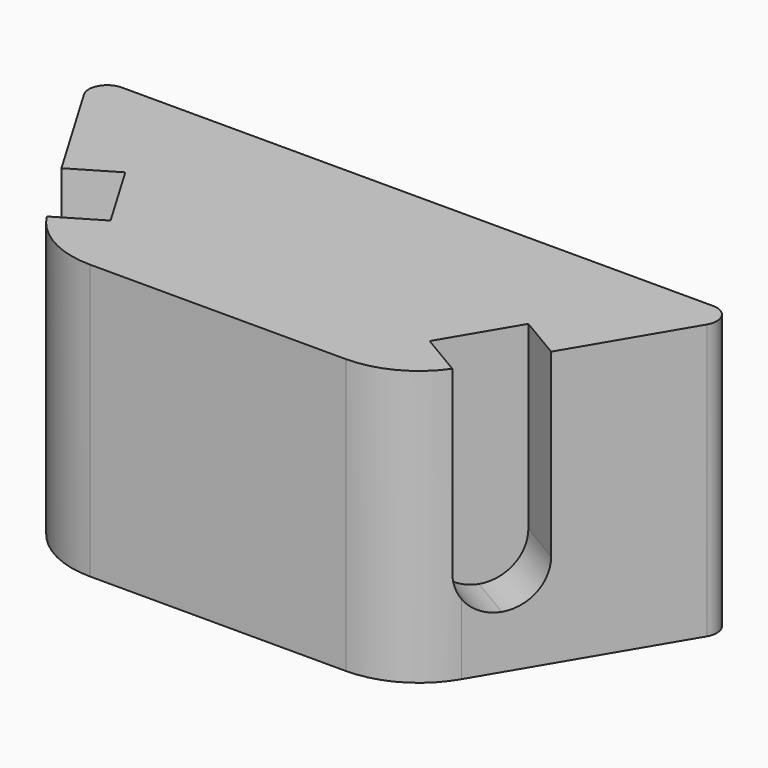
from build123d import *

# Parameters (mm, degrees)
F1_DEPTH = 30
F3_DEPTH = 24.2
F4_R     = 4.49999


# Not quite as in the source:
# - a fillet or chamfer is up to 0.001 mm smaller than in the source, because OpenCascade refuses the exact size


with BuildPart() as f1:
    # F0 (on Top) → F1 (new body)
    with BuildSketch(Plane.XY):
        with BuildLine():
            Line((-13.7223101757, 4.24), (14.2223098243, 4.24))
            ThreePointArc((14.2223098243, 4.24), (19.2223098243, 5.5797459622), (22.8825638622, 9.24))
            Line((22.8825638622, 9.24), (34.2739440306, 28.4706991862))
            ThreePointArc((34.2739440306, 28.4706991862), (34.2907944109, 30.4803025731), (32.5531808711, 31.49))
            Line((32.5531808711, 31.49), (-32.0531791289, 31.49))
            ThreePointArc((-32.0531791289, 31.49), (-33.7907926288, 30.4803026431), (-33.7739423706, 28.4706993249))
            Line((-33.7739423706, 28.4706993249), (-22.3825642135, 9.24))
            ThreePointArc((-22.3825642135, 9.24), (-18.7223101757, 5.5797459622), (-13.7223101757, 4.24))
        make_face()
    extrude(amount=F1_DEPTH)

    # F2 (on face) → F3 (cut)
    with BuildSketch(Plane.XY.offset(30)):
        with BuildLine():
            Line((-26.759759987, 16.6294953398), (-22.3825642135, 9.24))
            ThreePointArc((-22.3825642135, 9.24), (-22.2778836833, 9.0629195529), (-22.1695828196, 8.8880298132))
            Line((-22.1695828196, 8.8880298132), (-17.4408080346, 11.6891376089))
            Line((-17.4408080346, 11.6891376089), (-22.0276610725, 19.4325721963))
            Line((-22.0276610725, 19.4325721963), (-26.759759987, 16.6294953398))
        make_face()
        with BuildLine():
            Line((17.7215177836, 11.3189368702), (22.4312077057, 8.5291335532))
            ThreePointArc((22.4312077057, 8.5291335532), (22.6643714442, 8.879813846), (22.8825638622, 9.24))
            Line((22.8825638622, 9.24), (27.0404701341, 16.2592938501))
            Line((27.0404701341, 16.2592938501), (22.3083714455, 19.0623710879))
            Line((22.3083714455, 19.0623710879), (17.7215177836, 11.3189368702))
        make_face()
    extrude(amount=-F3_DEPTH, mode=Mode.SUBTRACT)

    # F4 (radius 4.5 in the source; OpenCascade refuses exactly that, so slightly less here)
    f4_edges = [f1.edges().sort_by_distance(p)[0] for p in [
        (-24.393711, 18.031034, 5.8),
        (-19.805195, 10.288584, 5.8),
        (24.674421, 17.660832, 5.8),
        (20.076363, 9.924035, 5.8),
    ]]
    fillet(f4_edges, radius=F4_R)


solid = f1.part
